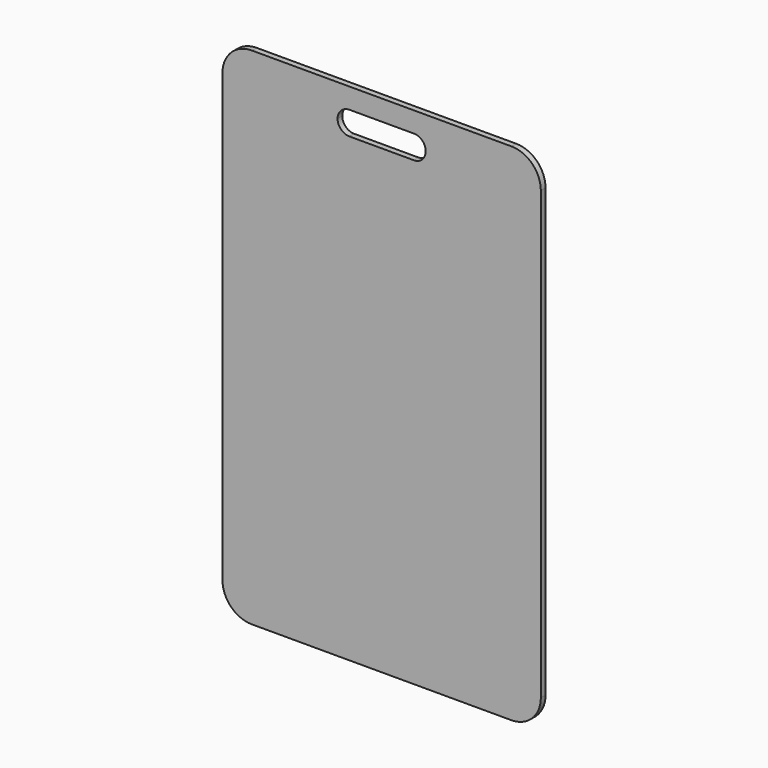
from build123d import *

# Parameters (mm, degrees)
F0_W     = 54.2
F0_H     = 86
F1_DEPTH = 1
F2_R     = 5
F3_R     = 1.99999


# Not quite as in the source:
# - a fillet or chamfer is up to 0.001 mm smaller than in the source, because OpenCascade refuses the exact size


with BuildPart() as f1:
    # F0 (on Front) → F1 (new body)
    with BuildSketch(Plane.XZ):
        Rectangle(F0_W, F0_H)
        Polygon((-7.5, 37.52), (-7.5, 39.52), (7.5, 39.52), (7.5, 37.52), (7.5, 35.52), (-7.5, 35.52), align=None, mode=Mode.SUBTRACT)
    extrude(amount=F1_DEPTH)

    # F2
    f2_edges = [f1.edges().sort_by_distance(p)[0] for p in [
        (-27.1, -0.5, 43),
        (27.1, -0.5, 43),
        (27.1, -0.5, -43),
        (-27.1, -0.5, -43),
    ]]
    fillet(f2_edges, radius=F2_R)

    # F3 (radius 2 in the source; OpenCascade refuses exactly that, so slightly less here)
    f3_edges = [f1.edges().sort_by_distance(p)[0] for p in [
        (-7.5, -0.5, 39.52),
        (-7.5, -0.5, 35.52),
        (7.5, -0.5, 35.52),
        (7.5, -0.5, 39.52),
    ]]
    fillet(f3_edges, radius=F3_R)


solid = f1.part
